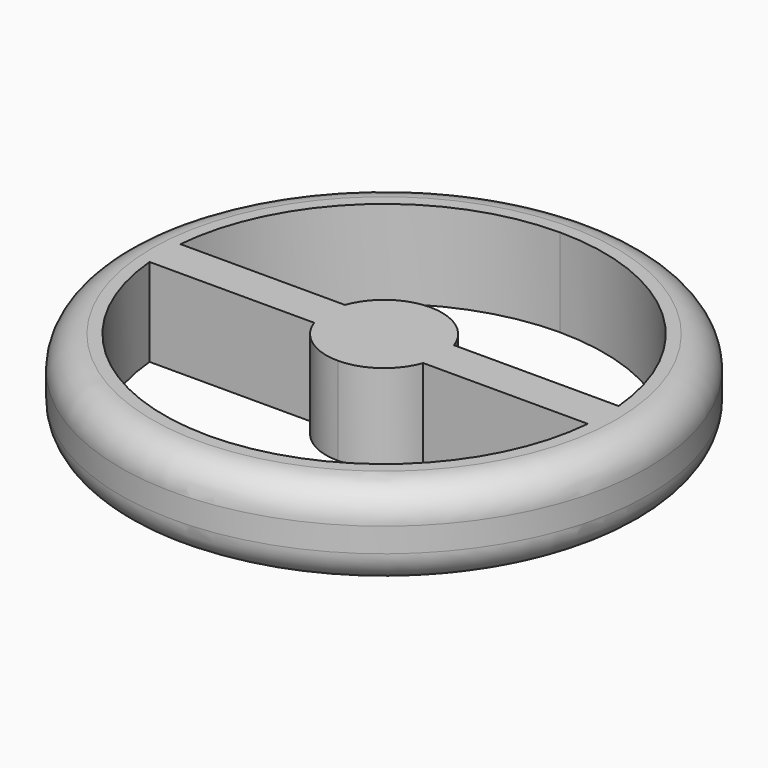
from build123d import *

# Parameters (mm, degrees)
F0_R     = 7.62
F1_DEPTH = 2.54
F2_R     = 0.9198153673


# Not quite as in the source:
# - a feature names something its author has since deleted; it is built from what else it names


with BuildPart() as f1:
    # F0 (on Top) → F1 (new body)
    with BuildSketch(Plane.XY):
        Circle(F0_R)
        with BuildLine():
            ThreePointArc((-6.325532194, -0.5569043569), (-6.3438800994, -0.2787207995), (-6.35, 0))
            ThreePointArc((-6.35, 0), (-6.3438800994, 0.2787207995), (-6.325532194, 0.5569043569))
            ThreePointArc((-6.325532194, 0.5569043569), (-4.28871527, 4.6828860047), (0, 6.35))
            ThreePointArc((0, 6.35), (4.28871527, 4.6828860047), (6.325532194, 0.5569043569))
            ThreePointArc((6.325532194, 0.5569043569), (6.3438800994, 0.2787207995), (6.35, 0))
            ThreePointArc((6.35, 0), (6.3438800994, -0.2787207995), (6.325532194, -0.5569043569))
            ThreePointArc((6.325532194, -0.5569043569), (4.28871527, -4.6828860047), (0, -6.35))
            ThreePointArc((0, -6.35), (-4.28871527, -4.6828860047), (-6.325532194, -0.5569043569))
        make_face(mode=Mode.SUBTRACT)
        with BuildLine():
            ThreePointArc((-1.5743877497, 0.5569043569), (-1.6459098023, 0.2825246393), (-1.6699818111, 0))
            Line((-1.6699818111, 0), (0, 0))
            Line((0, 0), (0, 0.5569043569))
            Line((0, 0.5569043569), (-1.5743877497, 0.5569043569))
        make_face()
        with BuildLine():
            ThreePointArc((-6.325532194, 0.5569043569), (-6.3438800994, 0.2787207995), (-6.35, 0))
            Line((-6.35, 0), (-1.6699818111, 0))
            ThreePointArc((-1.6699818111, 0), (-1.6459098023, 0.2825246393), (-1.5743877497, 0.5569043569))
            Line((-1.5743877497, 0.5569043569), (-6.325532194, 0.5569043569))
        make_face()
        with BuildLine():
            Line((-1.6699818111, 0), (-6.35, 0))
            ThreePointArc((-6.35, 0), (-6.3438800994, -0.2787207995), (-6.325532194, -0.5569043569))
            Line((-6.325532194, -0.5569043569), (-1.5743877497, -0.5569043569))
            ThreePointArc((-1.5743877497, -0.5569043569), (-1.6459098023, -0.2825246393), (-1.6699818111, 0))
        make_face()
        with BuildLine():
            Line((0, 0), (-1.6699818111, 0))
            ThreePointArc((-1.6699818111, 0), (-1.6459098023, -0.2825246393), (-1.5743877497, -0.5569043569))
            Line((-1.5743877497, -0.5569043569), (0, -0.5569043569))
            Line((0, -0.5569043569), (0, 0))
        make_face()
        with BuildLine():
            Line((0, 0.5569043569), (0, 0))
            Line((0, 0), (1.6699818111, 0))
            ThreePointArc((1.6699818111, 0), (1.6459098023, 0.2825246393), (1.5743877497, 0.5569043569))
            Line((1.5743877497, 0.5569043569), (0, 0.5569043569))
        make_face()
        with BuildLine():
            Line((1.5743877497, -0.5569043569), (6.325532194, -0.5569043569))
            ThreePointArc((6.325532194, -0.5569043569), (6.3438800994, -0.2787207995), (6.35, 0))
            Line((6.35, 0), (1.6699818111, 0))
            ThreePointArc((1.6699818111, 0), (1.6459098023, -0.2825246393), (1.5743877497, -0.5569043569))
        make_face()
        with BuildLine():
            Line((1.6699818111, 0), (0, 0))
            Line((0, 0), (0, -0.5569043569))
            Line((0, -0.5569043569), (1.5743877497, -0.5569043569))
            ThreePointArc((1.5743877497, -0.5569043569), (1.6459098023, -0.2825246393), (1.6699818111, 0))
        make_face()
        with BuildLine():
            ThreePointArc((1.5743877497, 0.5569043569), (0.9640588941, 1.3636090708), (0, 1.6699818111))
            Line((0, 1.6699818111), (0, 0.5569043569))
            Line((0, 0.5569043569), (1.5743877497, 0.5569043569))
        make_face()
        with BuildLine():
            ThreePointArc((0, 1.6699818111), (-0.9640588941, 1.3636090708), (-1.5743877497, 0.5569043569))
            Line((-1.5743877497, 0.5569043569), (0, 0.5569043569))
            Line((0, 0.5569043569), (0, 1.6699818111))
        make_face()
        with BuildLine():
            Line((0, -0.5569043569), (-1.5743877497, -0.5569043569))
            ThreePointArc((-1.5743877497, -0.5569043569), (-0.9640588941, -1.3636090708), (0, -1.6699818111))
            Line((0, -1.6699818111), (0, -0.5569043569))
        make_face()
        with BuildLine():
            Line((0, -0.5569043569), (0, -1.6699818111))
            ThreePointArc((0, -1.6699818111), (0.9640588941, -1.3636090708), (1.5743877497, -0.5569043569))
            Line((1.5743877497, -0.5569043569), (0, -0.5569043569))
        make_face()
        with BuildLine():
            ThreePointArc((6.35, 0), (6.3438800994, 0.2787207995), (6.325532194, 0.5569043569))
            Line((6.325532194, 0.5569043569), (1.5743877497, 0.5569043569))
            ThreePointArc((1.5743877497, 0.5569043569), (1.6459098023, 0.2825246393), (1.6699818111, 0))
            Line((1.6699818111, 0), (6.35, 0))
        make_face()
    extrude(amount=F1_DEPTH)

    # F2
    f2_edges = [f1.edges().sort_by_distance(p)[0] for p in [
        (-7.62, 0, 2.54),
        (-7.62, 0, 0),
    ]]
    fillet(f2_edges, radius=F2_R)


solid = f1.part
